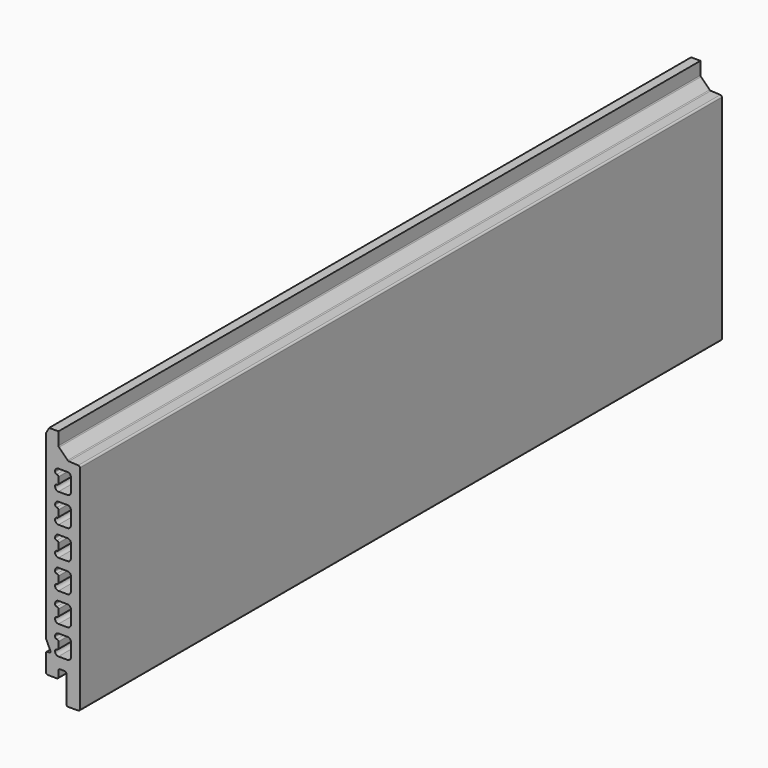
from build123d import *

# Parameters (mm, degrees)
F1_DEPTH = 711.2
F3_DEPTH = 711.2


# Not quite as in the source:
# - ends of sketch curves that miss each other by under 0.0002 mm in the source are joined


with BuildPart() as f1:
    # F0 (on Front) → F1 (new body)
    with BuildSketch(Plane.XZ):
        with BuildLine():
            ThreePointArc((-14.9999680608, -58.9985104), (-14.96444377, -59.322873513), (-14.8595551032, -59.6318585804))
            Line((-14.8595551032, -59.6318585804), (-11.0988328608, -67.6967912))
            ThreePointArc((-11.0988328608, -67.6967912), (-11.1617050028, -68.655791158), (-12.004294, -69.1180454046))
            Line((-12.004294, -69.1180454046), (-14.0009118, -69.1180736))
            ThreePointArc((-14.0009118, -69.1180736), (-14.707352628, -69.410690972), (-14.99997, -70.1171318))
            Line((-14.99997, -70.1171318), (-14.99997, -85.599397))
            ThreePointArc((-14.99997, -85.599397), (-14.5606310505, -86.6600550505), (-13.499973, -87.099394))
            Line((-13.499973, -87.099394), (-5.5003446, -87.099394))
            ThreePointArc((-5.5003446, -87.099394), (-4.4396865495, -86.6600550505), (-4.0003476, -85.599397))
            Line((-4.0003476, -85.599397), (-4.0003476, -80.5996356))
            ThreePointArc((-4.0003476, -80.5996356), (-3.5610086505, -79.5389775495), (-2.5003506, -79.0996386))
            Line((-2.5003506, -79.0996386), (1.4838426, -79.0996386))
            ThreePointArc((1.4838426, -79.0996386), (2.5445365709, -79.5390134712), (2.9838395966, -80.5997372))
            Line((2.9838395966, -80.5997372), (2.98196, -104.5986224))
            ThreePointArc((2.98196, -104.5986224), (3.4212540492, -105.6593625482), (4.481957, -106.0987464))
            Line((4.481957, -106.0987464), (13.499973, -106.0987464))
            ThreePointArc((13.499973, -106.0987464), (14.5606310505, -105.6594074505), (14.99997, -104.5987494))
            Line((14.99997, -104.5987494), (14.99997, 83.7761342))
            ThreePointArc((14.99997, 83.7761342), (14.5844487053, 84.8124273268), (13.5680958768, 85.2745834897))
            Line((13.5680958768, 85.2745834897), (5.104384, 85.6592902))
            ThreePointArc((5.104384, 85.6592902), (4.5671403109, 85.7853117853), (4.1118233495, 86.0970797495))
            Line((4.1118233495, 86.0970797495), (-3.5610038, 93.7699166))
            ThreePointArc((-3.5610038, 93.7699166), (-3.8861671271, 94.2565457995), (-4.0003476, 94.8305698))
            Line((-4.0003476, 94.8305698), (-4.0003476, 106.0987464))
            Line((-4.0003476, 106.0987464), (-12.3105164, 106.0987464))
            Line((-12.3105164, 106.0987464), (-14.99997, 101.2086876))
            Line((-14.99997, 101.2086876), (-14.9999680608, -58.9985104))
        make_face()
    extrude(amount=F1_DEPTH)

    # F2 (on Front) → F3 (cut)
    with BuildSketch(Plane.XZ):
        with BuildLine():
            ThreePointArc((-5.49529, -31.195264), (-4.4346319495, -31.6346029495), (-3.995293, -32.695261))
            Line((-3.995293, -32.695261), (-3.995293, -37.695251))
            ThreePointArc((-3.995293, -37.695251), (-4.4346319495, -38.7559090505), (-5.49529, -39.195248))
            Line((-5.49529, -39.195248), (-5.499989, -39.195248))
            ThreePointArc((-5.499989, -39.195248), (-6.5606470505, -39.6345869495), (-6.999986, -40.695245))
            Line((-6.999986, -40.695245), (-6.999986, -41.195244))
            ThreePointArc((-6.999986, -41.195244), (-6.1213081009, -43.3165601009), (-3.999992, -44.195238))
            Line((-3.999992, -44.195238), (3.999992, -44.195238))
            ThreePointArc((3.999992, -44.195238), (6.1213081009, -43.3165601009), (6.999986, -41.195244))
            Line((6.999986, -41.195244), (6.999986, -29.195268))
            ThreePointArc((6.999986, -29.195268), (6.1213081009, -27.0739518991), (3.999992, -26.195274))
            Line((3.999992, -26.195274), (-3.999992, -26.195274))
            ThreePointArc((-3.999992, -26.195274), (-6.1213081009, -27.0739518991), (-6.999986, -29.195268))
            Line((-6.999986, -29.195268), (-6.999986, -29.695267))
            ThreePointArc((-6.999986, -29.695267), (-6.5606470505, -30.7559250505), (-5.499989, -31.195264))
            Line((-5.499989, -31.195264), (-5.49529, -31.195264))
        make_face()
        with BuildLine():
            ThreePointArc((-5.49529, -56.595264), (-4.4346319495, -57.0346029495), (-3.995293, -58.095261))
            Line((-3.995293, -58.095261), (-3.995293, -63.095251))
            ThreePointArc((-3.995293, -63.095251), (-4.4346319495, -64.1559090505), (-5.49529, -64.595248))
            Line((-5.49529, -64.595248), (-5.499989, -64.595248))
            ThreePointArc((-5.499989, -64.595248), (-6.5606470505, -65.0345869495), (-6.999986, -66.095245))
            Line((-6.999986, -66.095245), (-6.999986, -66.595244))
            ThreePointArc((-6.999986, -66.595244), (-6.1213081009, -68.7165601009), (-3.999992, -69.595238))
            Line((-3.999992, -69.595238), (0, -69.595238))
            Line((0, -69.595238), (3.999992, -69.595238))
            ThreePointArc((3.999992, -69.595238), (6.1213081009, -68.7165601009), (6.999986, -66.595244))
            Line((6.999986, -66.595244), (6.999986, -54.595268))
            ThreePointArc((6.999986, -54.595268), (6.1213081009, -52.4739518991), (3.999992, -51.595274))
            Line((3.999992, -51.595274), (-3.999992, -51.595274))
            ThreePointArc((-3.999992, -51.595274), (-6.1213081009, -52.4739518991), (-6.999986, -54.595268))
            Line((-6.999986, -54.595268), (-6.999986, -55.095267))
            ThreePointArc((-6.999986, -55.095267), (-6.5606470505, -56.1559250505), (-5.499989, -56.595264))
            Line((-5.499989, -56.595264), (-5.49529, -56.595264))
        make_face()
        with BuildLine():
            ThreePointArc((-5.49529, -5.3953664), (-4.4346319495, -5.8347053495), (-3.995293, -6.8953634))
            Line((-3.995293, -6.8953634), (-3.995293, -11.8953534))
            ThreePointArc((-3.995293, -11.8953534), (-4.4346319495, -12.9560114505), (-5.49529, -13.3953504))
            Line((-5.49529, -13.3953504), (-5.499989, -13.3953504))
            ThreePointArc((-5.499989, -13.3953504), (-6.5606470505, -13.8346893495), (-6.999986, -14.8953474))
            Line((-6.999986, -14.8953474), (-6.999986, -15.3953464))
            ThreePointArc((-6.999986, -15.3953464), (-6.1213081009, -17.5166625009), (-3.999992, -18.3953404))
            Line((-3.999992, -18.3953404), (3.999992, -18.3953404))
            ThreePointArc((3.999992, -18.3953404), (6.1213081009, -17.5166625009), (6.999986, -15.3953464))
            Line((6.999986, -15.3953464), (6.999986, -3.3953704))
            ThreePointArc((6.999986, -3.3953704), (6.1213081009, -1.2740542991), (3.999992, -0.3953764))
            Line((3.999992, -0.3953764), (-3.999992, -0.3953764))
            ThreePointArc((-3.999992, -0.3953764), (-6.1213081009, -1.2740542991), (-6.999986, -3.3953704))
            Line((-6.999986, -3.3953704), (-6.999986, -3.8953694))
            ThreePointArc((-6.999986, -3.8953694), (-6.5606470505, -4.9560274505), (-5.499989, -5.3953664))
            Line((-5.499989, -5.3953664), (-5.49529, -5.3953664))
        make_face()
        with BuildLine():
            Line((-5.499989, 20.4015086), (-5.49529, 20.4015086))
            ThreePointArc((-5.49529, 20.4015086), (-4.4346319495, 19.9621696505), (-3.995293, 18.9015116))
            Line((-3.995293, 18.9015116), (-3.995293, 13.9015216))
            ThreePointArc((-3.995293, 13.9015216), (-4.4346319495, 12.8408635495), (-5.49529, 12.4015246))
            Line((-5.49529, 12.4015246), (-5.499989, 12.4015246))
            ThreePointArc((-5.499989, 12.4015246), (-6.5606470505, 11.9621856505), (-6.999986, 10.9015276))
            Line((-6.999986, 10.9015276), (-6.999986, 10.4015286))
            ThreePointArc((-6.999986, 10.4015286), (-6.1213081009, 8.2802124991), (-3.999992, 7.4015346))
            Line((-3.999992, 7.4015346), (3.999992, 7.4015346))
            ThreePointArc((3.999992, 7.4015346), (6.1213081009, 8.2802124991), (6.999986, 10.4015286))
            Line((6.999986, 10.4015286), (6.999986, 22.4015046))
            ThreePointArc((6.999986, 22.4015046), (6.1213081009, 24.5228207009), (3.999992, 25.4014986))
            Line((3.999992, 25.4014986), (-3.999992, 25.4014986))
            ThreePointArc((-3.999992, 25.4014986), (-6.1213081009, 24.5228207009), (-6.999986, 22.4015046))
            Line((-6.999986, 22.4015046), (-6.999986, 21.9015056))
            ThreePointArc((-6.999986, 21.9015056), (-6.5606470505, 20.8408475495), (-5.499989, 20.4015086))
        make_face()
        with BuildLine():
            Line((-5.499989, 46.1983836), (-5.49529, 46.1983836))
            ThreePointArc((-5.49529, 46.1983836), (-4.4346319495, 45.7590446505), (-3.995293, 44.6983866))
            Line((-3.995293, 44.6983866), (-3.995293, 39.6983966))
            ThreePointArc((-3.995293, 39.6983966), (-4.4346319495, 38.6377385495), (-5.49529, 38.1983996))
            Line((-5.49529, 38.1983996), (-5.499989, 38.1983996))
            ThreePointArc((-5.499989, 38.1983996), (-6.5606470505, 37.7590606505), (-6.999986, 36.6984026))
            Line((-6.999986, 36.6984026), (-6.999986, 36.1984036))
            ThreePointArc((-6.999986, 36.1984036), (-6.1213081009, 34.0770874991), (-3.999992, 33.1984096))
            Line((-3.999992, 33.1984096), (3.999992, 33.1984096))
            ThreePointArc((3.999992, 33.1984096), (6.1213081009, 34.0770874991), (6.999986, 36.1984036))
            Line((6.999986, 36.1984036), (6.999986, 48.1983796))
            ThreePointArc((6.999986, 48.1983796), (6.1213081009, 50.3196957009), (3.999992, 51.1983736))
            Line((3.999992, 51.1983736), (-3.999992, 51.1983736))
            ThreePointArc((-3.999992, 51.1983736), (-6.1213081009, 50.3196957009), (-6.999986, 48.1983796))
            Line((-6.999986, 48.1983796), (-6.999986, 47.6983806))
            ThreePointArc((-6.999986, 47.6983806), (-6.5606470505, 46.6377225495), (-5.499989, 46.1983836))
        make_face()
        with BuildLine():
            Line((-5.499989, 71.9952586), (-5.49529, 71.9952586))
            ThreePointArc((-5.49529, 71.9952586), (-4.4346319495, 71.5559196505), (-3.995293, 70.4952616))
            Line((-3.995293, 70.4952616), (-3.995293, 65.4952716))
            ThreePointArc((-3.995293, 65.4952716), (-4.4346319495, 64.4346135495), (-5.49529, 63.9952746))
            Line((-5.49529, 63.9952746), (-5.499989, 63.9952746))
            ThreePointArc((-5.499989, 63.9952746), (-6.5606470505, 63.5559356505), (-6.999986, 62.4952776))
            Line((-6.999986, 62.4952776), (-6.999986, 61.9952786))
            ThreePointArc((-6.999986, 61.9952786), (-6.1213081009, 59.8739624991), (-3.999992, 58.9952846))
            Line((-3.999992, 58.9952846), (3.999992, 58.9952846))
            ThreePointArc((3.999992, 58.9952846), (6.1213081009, 59.8739624991), (6.999986, 61.9952786))
            Line((6.999986, 61.9952786), (6.999986, 73.9952546))
            ThreePointArc((6.999986, 73.9952546), (6.1213081009, 76.1165707009), (3.999992, 76.9952486))
            Line((3.999992, 76.9952486), (-3.999992, 76.9952486))
            ThreePointArc((-3.999992, 76.9952486), (-6.1213081009, 76.1165707009), (-6.999986, 73.9952546))
            Line((-6.999986, 73.9952546), (-6.999986, 73.4952556))
            ThreePointArc((-6.999986, 73.4952556), (-6.5606470505, 72.4345975495), (-5.499989, 71.9952586))
        make_face()
    extrude(amount=F3_DEPTH, mode=Mode.SUBTRACT)


solid = f1.part
